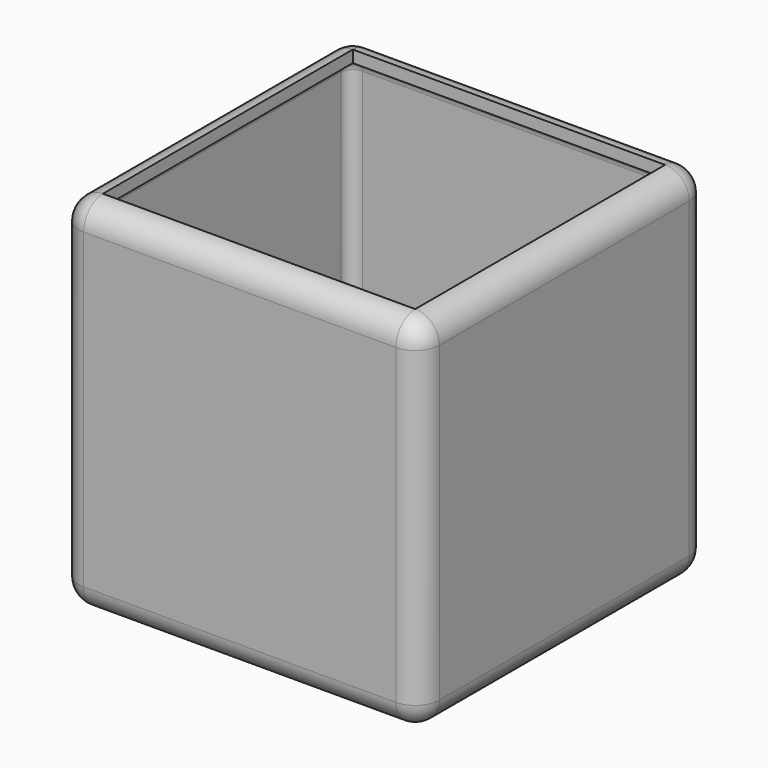
from build123d import *

# Parameters (mm, degrees)
F0_W     = 76.2
F0_H     = 76.2
F1_DEPTH = 38.1
F2_R     = 5.08
F3_T     = -2.54


# Not quite as in the source:
# - a shell that OpenCascade refuses in one call is made with other operations: the cavity is built on its own and cut out


with BuildPart() as f1:
    # F0 (on Front) → F1 (new body, symmetric)
    with BuildSketch(Plane.XZ):
        Rectangle(F0_W, F0_H)
    extrude(amount=F1_DEPTH, both=True)

    # F2
    f2_edges = [f1.edges().sort_by_distance(p)[0] for p in [
        (0, 38.1, 38.1),
        (-38.1, 0, 38.1),
        (0, -38.1, 38.1),
        (38.1, 0, 38.1),
        (38.1, 38.1, 0),
        (38.1, -38.1, 0),
        (38.1, 0, -38.1),
        (-38.1, -38.1, 0),
        (0, -38.1, -38.1),
        (-38.1, 0, -38.1),
        (0, 38.1, -38.1),
        (-38.1, 38.1, 0),
    ]]
    fillet(f2_edges, radius=F2_R)

    # F3: a shell. OpenCascade refuses it in one call, so the cavity is built on its own and cut out:
    # the body offset inwards by the wall thickness, plus a prism from it out through each open face.
    f3_core = offset(f1.part, amount=F3_T, mode=Mode.PRIVATE)
    f3_exits = [f3_core.faces().sort_by_distance(p)[0] for p in [
        (0, 0, 35.56),
    ]]
    add(f3_core, mode=Mode.SUBTRACT)
    extrude(f3_exits, amount=-F3_T, mode=Mode.SUBTRACT)


solid = f1.part
